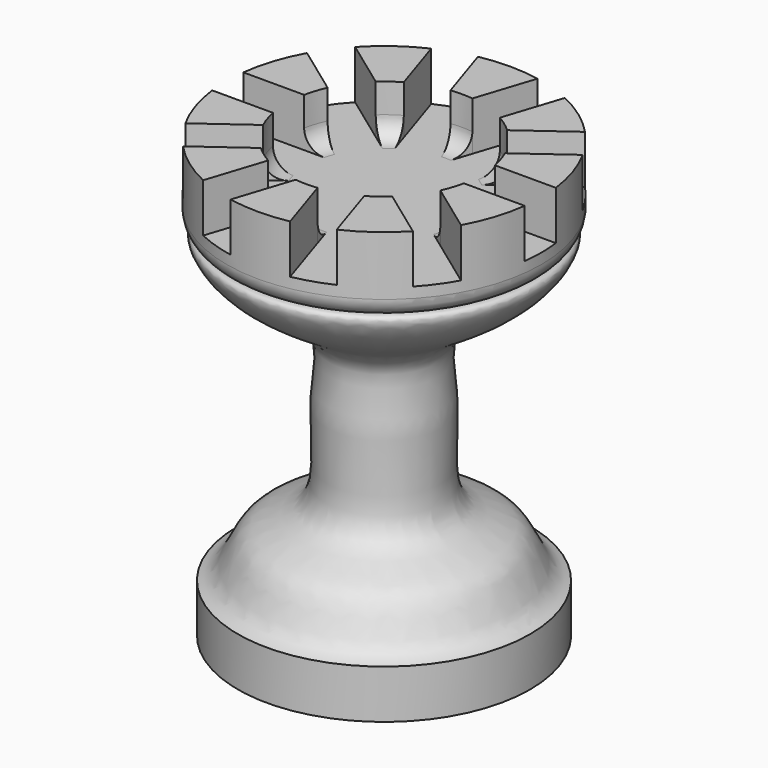
from build123d import *

# Parameters (mm, degrees)
F2_R          = 12.7
F3_DEPTH      = 6.35
F4_W          = 13.9516657994
F4_H          = 5.08
F5_DEPTH      = 6.35
F6_T4_ANGLE   = 70.2223360854
F6_T9_ANGLE   = 70.2223360854
F6_T15_ANGLE  = 70.2223360854
F6_T20_ANGLE  = 70.2223360854
F6_T25_ANGLE  = 70.2223360854
F6_T31_ANGLE  = 70.2223360854
F6_T36_ANGLE  = 70.2223360854
F6_T41_ANGLE  = 70.2223360854
F6_T47_ANGLE  = 70.2223360854
F6_T52_ANGLE  = 70.2223360854
F6_T57_ANGLE  = 70.2223360854
F6_T63_ANGLE  = 70.2223360854
F6_T68_ANGLE  = 70.2223360854
F6_T73_ANGLE  = 70.2223360854
F6_T79_ANGLE  = 70.2223360854
F6_T84_ANGLE  = 70.2223360854
F6_T89_ANGLE  = 70.2223360854
F6_T95_ANGLE  = 70.2223360854
F6_T100_ANGLE = 70.2223360854
F6_T105_ANGLE = 70.2223360854
F6_T111_ANGLE = 70.2223360854
F6_T116_ANGLE = 70.2223360854
F6_T121_ANGLE = 70.2223360854
F6_T127_ANGLE = 70.2223360854
F6_T132_ANGLE = 70.2223360854
F6_T137_ANGLE = 70.2223360854
F6_T143_ANGLE = 70.2223360854
F6_T148_ANGLE = 70.2223360854
F6_T153_ANGLE = 70.2223360854
F6_T159_ANGLE = 70.2223360854


# Not quite as in the source:
# - a fillet or chamfer that OpenCascade refuses, or shapes differently, is made with other operations: its cross-section is extruded or revolved along the edge and cut away or added


with BuildPart() as f1:
    # F0 (on Front) → F1 (revolve)
    with BuildSketch(Plane.XZ):
        Polygon((0, 56.9858625531), (0, 46.99), (19.1146062934, 46.99), (20.5274569789, 46.99), (20.5274569789, 56.9858625531), align=None)
        with BuildLine():
            Line((0, 46.99), (0, 0))
            Line((0, 0), (19.05, 0))
            Line((19.05, 0), (19.05, 6.35))
            add(Edge.make_bspline(
                [(19.05, 6.35), (16.5339762391, 6.9432851518), (16.0569680771, 13.155913981), (7.6273097689, 13.9182189792), (7.2848350223, 21.1697275176), (7.7653617057, 27.9522467214), (6.3029058207, 34.9075424246), (11.924104766, 38.4900940868), (18.9862936416, 42.8343809655), (20.5274569789, 46.99), (19.1146062934, 46.99)],
                knots=[0, 0, 0, 0, 0.1315490965, 0.2608144657, 0.383337474, 0.5182610911, 0.6426548645, 0.7643816563, 0.9167734046, 1, 1, 1, 1], degree=3))
            Line((19.1146062934, 46.99), (0, 46.99))
        make_face()
    revolve(axis=Axis((0, 0, 28.575), (0, 0, 1)))

    # F2 (on face) → F3 (cut)
    with BuildSketch(Plane.XY.offset(56.9858625531)):
        Circle(F2_R)
    extrude(amount=-F3_DEPTH, mode=Mode.SUBTRACT)

    # F4 (on face) → F5 (cut)
    with BuildSketch(Plane.XY.offset(56.9858625531)):
        with Locations((15.748, 0)):
            Rectangle(F4_W, F4_H)
        Polygon((8.5898068025, 3.1012472865), (19.876941534, 11.3018306883), (16.8909924524, 15.4116370197), (5.6038577208, 7.2110536179), align=None)
        Polygon((5.1264322629, 7.5579235171), (9.4377340947, 20.8267461887), (4.606366992, 22.3965525202), (0.2950651601, 9.1277298485), align=None)
        Polygon((-0.2950651601, 9.1277298485), (-4.606366992, 22.3965525202), (-9.4377340947, 20.8267461887), (-5.1264322629, 7.5579235171), align=None)
        Polygon((-5.6038577208, 7.2110536179), (-16.8909924524, 15.4116370197), (-19.876941534, 11.3018306883), (-8.5898068025, 3.1012472865), align=None)
        with Locations((-15.748, 0)):
            Rectangle(F4_W, F4_H)
        Polygon((-8.5898068025, -3.1012472865), (-19.876941534, -11.3018306883), (-16.8909924524, -15.4116370197), (-5.6038577208, -7.2110536179), align=None)
        Polygon((-5.1264322629, -7.5579235171), (-9.4377340947, -20.8267461887), (-4.606366992, -22.3965525202), (-0.2950651601, -9.1277298485), align=None)
        Polygon((0.2950651601, -9.1277298485), (4.606366992, -22.3965525202), (9.4377340947, -20.8267461887), (5.1264322629, -7.5579235171), align=None)
        Polygon((5.6038577208, -7.2110536179), (16.8909924524, -15.4116370197), (19.876941534, -11.3018306883), (8.5898068025, -3.1012472865), align=None)
    extrude(amount=-F5_DEPTH, mode=Mode.SUBTRACT)

    # F6: fillet of radius 2.54 on 11 edges, made by hand


with BuildPart() as f6_tool2:
    # F6_s3 → F6_t4 (revolve)
    with BuildSketch(Plane(origin=(0, 0, 0), x_dir=(0, 0, 1), z_dir=(-0.3237330019, 0.9461484786, 0))):
        with BuildLine():
            ThreePointArc((50.6358625531, -10.16), (51.3798113289, -11.9560512242), (53.1758625531, -12.7))
            Line((53.1758625531, -12.7), (50.6358625531, -12.7))
            Line((50.6358625531, -12.7), (50.6358625531, -10.16))
        make_face()
    revolve(axis=Axis((0, 0, 50.6358625531), (0, 0, 1)), revolution_arc=F6_T4_ANGLE)

    split(bisect_by=Plane(origin=(-1.4929745408, 2.0549031657, 0), x_dir=(0, 0, 1), z_dir=(-0.5877852523, 0.8090169944, 0)), keep=Keep.TOP)


with BuildPart() as f1_1:
    add(f1.part)

    # F6_t1: union F6_tool2
    add(f6_tool2.part)


with BuildPart() as f6_tool7:
    # F6_s8 → F6_t9 (revolve)
    with BuildSketch(Plane(origin=(0, 0, 0), x_dir=(0, 0, 1), z_dir=(-0.3237330019, 0.9461484786, 0))):
        with BuildLine():
            ThreePointArc((50.6358625531, -10.16), (51.3798113289, -11.9560512242), (53.1758625531, -12.7))
            Line((53.1758625531, -12.7), (50.6358625531, -12.7))
            Line((50.6358625531, -12.7), (50.6358625531, -10.16))
        make_face()
    revolve(axis=Axis((0, 0, 50.6358625531), (0, 0, 1)), revolution_arc=F6_T9_ANGLE)

    split(bisect_by=Plane(origin=(1.4929745408, -2.0549031657, 0), x_dir=(0, 0, 1), z_dir=(0.5877852523, -0.8090169944, 0)), keep=Keep.TOP)

    split(bisect_by=Plane(origin=(-2.4156835514, 0.7849031657, 0), x_dir=(0, 0, 1), z_dir=(-0.9510565163, 0.3090169944, 0)), keep=Keep.TOP)


with BuildPart() as f1_2:
    add(f1_1.part)

    # F6_t6: union F6_tool7
    add(f6_tool7.part)


with BuildPart() as f6_tool13:
    # F6_s14 → F6_t15 (revolve)
    with BuildSketch(Plane(origin=(0, 0, 0), x_dir=(0, 0, 1), z_dir=(-0.3237330019, 0.9461484786, 0))):
        with BuildLine():
            ThreePointArc((50.6358625531, -10.16), (51.3798113289, -11.9560512242), (53.1758625531, -12.7))
            Line((53.1758625531, -12.7), (50.6358625531, -12.7))
            Line((50.6358625531, -12.7), (50.6358625531, -10.16))
        make_face()
    revolve(axis=Axis((0, 0, 50.6358625531), (0, 0, 1)), revolution_arc=F6_T15_ANGLE)

    split(bisect_by=Plane(origin=(2.4156835514, -0.7849031657, 0), x_dir=(0, 0, 1), z_dir=(0.9510565163, -0.3090169944, 0)), keep=Keep.TOP)


with BuildPart() as f1_3:
    add(f1_2.part)

    # F6_t12: union F6_tool13
    add(f6_tool13.part)


with BuildPart() as f6_tool18:
    # F6_s19 → F6_t20 (revolve)
    with BuildSketch(Plane(origin=(0, 0, 0), x_dir=(0, 0, 1), z_dir=(0.294226622, 0.9557356826, 0))):
        with BuildLine():
            ThreePointArc((50.6358625531, -10.16), (51.3798113289, -11.9560512242), (53.1758625531, -12.7))
            Line((53.1758625531, -12.7), (50.6358625531, -12.7))
            Line((50.6358625531, -12.7), (50.6358625531, -10.16))
        make_face()
    revolve(axis=Axis((0, 0, 50.6358625531), (0, 0, 1)), revolution_arc=F6_T20_ANGLE)

    split(bisect_by=Plane.XZ.offset(-2.54), keep=Keep.BOTTOM)


with BuildPart() as f1_4:
    add(f1_3.part)

    # F6_t17: union F6_tool18
    add(f6_tool18.part)


with BuildPart() as f6_tool23:
    # F6_s24 → F6_t25 (revolve)
    with BuildSketch(Plane(origin=(0, 0, 0), x_dir=(0, 0, 1), z_dir=(0.294226622, 0.9557356826, 0))):
        with BuildLine():
            ThreePointArc((50.6358625531, -10.16), (51.3798113289, -11.9560512242), (53.1758625531, -12.7))
            Line((53.1758625531, -12.7), (50.6358625531, -12.7))
            Line((50.6358625531, -12.7), (50.6358625531, -10.16))
        make_face()
    revolve(axis=Axis((0, 0, 50.6358625531), (0, 0, 1)), revolution_arc=F6_T25_ANGLE)

    split(bisect_by=Plane.XZ.offset(2.54), keep=Keep.TOP)

    split(bisect_by=Plane(origin=(-1.4929745408, 2.0549031657, 0), x_dir=(0, 0, 1), z_dir=(-0.5877852523, 0.8090169944, 0)), keep=Keep.TOP)


with BuildPart() as f1_5:
    add(f1_4.part)

    # F6_t22: union F6_tool23
    add(f6_tool23.part)


with BuildPart() as f6_tool29:
    # F6_s30 → F6_t31 (revolve)
    with BuildSketch(Plane(origin=(0, 0, 0), x_dir=(0, 0, 1), z_dir=(0.294226622, 0.9557356826, 0))):
        with BuildLine():
            ThreePointArc((50.6358625531, -10.16), (51.3798113289, -11.9560512242), (53.1758625531, -12.7))
            Line((53.1758625531, -12.7), (50.6358625531, -12.7))
            Line((50.6358625531, -12.7), (50.6358625531, -10.16))
        make_face()
    revolve(axis=Axis((0, 0, 50.6358625531), (0, 0, 1)), revolution_arc=F6_T31_ANGLE)

    split(bisect_by=Plane(origin=(1.4929745408, -2.0549031657, 0), x_dir=(0, 0, 1), z_dir=(0.5877852523, -0.8090169944, 0)), keep=Keep.TOP)


with BuildPart() as f1_6:
    add(f1_5.part)

    # F6_t28: union F6_tool29
    add(f6_tool29.part)


with BuildPart() as f6_tool34:
    # F6_s35 → F6_t36 (revolve)
    with BuildSketch(Plane(origin=(0, 0, 0), x_dir=(0, 0, 1), z_dir=(0.7998016767, 0.6002643401, 0))):
        with BuildLine():
            ThreePointArc((50.6358625531, -10.16), (51.3798113289, -11.9560512242), (53.1758625531, -12.7))
            Line((53.1758625531, -12.7), (50.6358625531, -12.7))
            Line((50.6358625531, -12.7), (50.6358625531, -10.16))
        make_face()
    revolve(axis=Axis((0, 0, 50.6358625531), (0, 0, 1)), revolution_arc=F6_T36_ANGLE)

    split(bisect_by=Plane(origin=(1.4929745408, 2.0549031657, 0), x_dir=(0, 0, 1), z_dir=(0.5877852523, 0.8090169944, 0)), keep=Keep.TOP)


with BuildPart() as f1_7:
    add(f1_6.part)

    # F6_t33: union F6_tool34
    add(f6_tool34.part)


with BuildPart() as f6_tool39:
    # F6_s40 → F6_t41 (revolve)
    with BuildSketch(Plane(origin=(0, 0, 0), x_dir=(0, 0, 1), z_dir=(0.7998016767, 0.6002643401, 0))):
        with BuildLine():
            ThreePointArc((50.6358625531, -10.16), (51.3798113289, -11.9560512242), (53.1758625531, -12.7))
            Line((53.1758625531, -12.7), (50.6358625531, -12.7))
            Line((50.6358625531, -12.7), (50.6358625531, -10.16))
        make_face()
    revolve(axis=Axis((0, 0, 50.6358625531), (0, 0, 1)), revolution_arc=F6_T41_ANGLE)

    split(bisect_by=Plane(origin=(-1.4929745408, -2.0549031657, 0), x_dir=(0, 0, 1), z_dir=(-0.5877852523, -0.8090169944, 0)), keep=Keep.TOP)

    split(bisect_by=Plane.XZ.offset(-2.54), keep=Keep.BOTTOM)


with BuildPart() as f1_8:
    add(f1_7.part)

    # F6_t38: union F6_tool39
    add(f6_tool39.part)


with BuildPart() as f6_tool45:
    # F6_s46 → F6_t47 (revolve)
    with BuildSketch(Plane(origin=(0, 0, 0), x_dir=(0, 0, 1), z_dir=(0.7998016767, 0.6002643401, 0))):
        with BuildLine():
            ThreePointArc((50.6358625531, -10.16), (51.3798113289, -11.9560512242), (53.1758625531, -12.7))
            Line((53.1758625531, -12.7), (50.6358625531, -12.7))
            Line((50.6358625531, -12.7), (50.6358625531, -10.16))
        make_face()
    revolve(axis=Axis((0, 0, 50.6358625531), (0, 0, 1)), revolution_arc=F6_T47_ANGLE)

    split(bisect_by=Plane.XZ.offset(2.54), keep=Keep.TOP)


with BuildPart() as f1_9:
    add(f1_8.part)

    # F6_t44: union F6_tool45
    add(f6_tool45.part)


with BuildPart() as f6_tool50:
    # F6_s51 → F6_t52 (revolve)
    with BuildSketch(Plane(origin=(0, 0, 0), x_dir=(0, 0, 1), z_dir=(-0.8180376224, 0.5751647141, 0))):
        with BuildLine():
            ThreePointArc((50.6358625531, -10.16), (51.3798113289, -11.9560512242), (53.1758625531, -12.7))
            Line((53.1758625531, -12.7), (50.6358625531, -12.7))
            Line((50.6358625531, -12.7), (50.6358625531, -10.16))
        make_face()
    revolve(axis=Axis((0, 0, 50.6358625531), (0, 0, 1)), revolution_arc=F6_T52_ANGLE)

    split(bisect_by=Plane(origin=(-2.4156835514, 0.7849031657, 0), x_dir=(0, 0, 1), z_dir=(-0.9510565163, 0.3090169944, 0)), keep=Keep.TOP)


with BuildPart() as f1_10:
    add(f1_9.part)

    # F6_t49: union F6_tool50
    add(f6_tool50.part)


with BuildPart() as f6_tool55:
    # F6_s56 → F6_t57 (revolve)
    with BuildSketch(Plane(origin=(0, 0, 0), x_dir=(0, 0, 1), z_dir=(-0.8180376224, 0.5751647141, 0))):
        with BuildLine():
            ThreePointArc((50.6358625531, -10.16), (51.3798113289, -11.9560512242), (53.1758625531, -12.7))
            Line((53.1758625531, -12.7), (50.6358625531, -12.7))
            Line((50.6358625531, -12.7), (50.6358625531, -10.16))
        make_face()
    revolve(axis=Axis((0, 0, 50.6358625531), (0, 0, 1)), revolution_arc=F6_T57_ANGLE)

    split(bisect_by=Plane(origin=(2.4156835514, -0.7849031657, 0), x_dir=(0, 0, 1), z_dir=(0.9510565163, -0.3090169944, 0)), keep=Keep.TOP)

    split(bisect_by=Plane(origin=(-2.4156835514, -0.7849031657, 0), x_dir=(0, 0, 1), z_dir=(-0.9510565163, -0.3090169944, 0)), keep=Keep.TOP)


with BuildPart() as f1_11:
    add(f1_10.part)

    # F6_t54: union F6_tool55
    add(f6_tool55.part)


with BuildPart() as f6_tool61:
    # F6_s62 → F6_t63 (revolve)
    with BuildSketch(Plane(origin=(0, 0, 0), x_dir=(0, 0, 1), z_dir=(-0.8180376224, 0.5751647141, 0))):
        with BuildLine():
            ThreePointArc((50.6358625531, -10.16), (51.3798113289, -11.9560512242), (53.1758625531, -12.7))
            Line((53.1758625531, -12.7), (50.6358625531, -12.7))
            Line((50.6358625531, -12.7), (50.6358625531, -10.16))
        make_face()
    revolve(axis=Axis((0, 0, 50.6358625531), (0, 0, 1)), revolution_arc=F6_T63_ANGLE)

    split(bisect_by=Plane(origin=(2.4156835514, 0.7849031657, 0), x_dir=(0, 0, 1), z_dir=(0.9510565163, 0.3090169944, 0)), keep=Keep.TOP)


with BuildPart() as f1_12:
    add(f1_11.part)

    # F6_t60: union F6_tool61
    add(f6_tool61.part)


with BuildPart() as f6_tool66:
    # F6_s67 → F6_t68 (revolve)
    with BuildSketch(Plane(origin=(0, 0, 0), x_dir=(0, 0, 1), z_dir=(-0.9998796751, -0.0155124219, 0))):
        with BuildLine():
            ThreePointArc((50.6358625531, -10.16), (51.3798113289, -11.9560512242), (53.1758625531, -12.7))
            Line((53.1758625531, -12.7), (50.6358625531, -12.7))
            Line((50.6358625531, -12.7), (50.6358625531, -10.16))
        make_face()
    revolve(axis=Axis((0, 0, 50.6358625531), (0, 0, 1)), revolution_arc=F6_T68_ANGLE)

    split(bisect_by=Plane(origin=(-2.4156835514, -0.7849031657, 0), x_dir=(0, 0, 1), z_dir=(-0.9510565163, -0.3090169944, 0)), keep=Keep.TOP)


with BuildPart() as f1_13:
    add(f1_12.part)

    # F6_t65: union F6_tool66
    add(f6_tool66.part)


with BuildPart() as f6_tool71:
    # F6_s72 → F6_t73 (revolve)
    with BuildSketch(Plane(origin=(0, 0, 0), x_dir=(0, 0, 1), z_dir=(-0.9998796751, -0.0155124219, 0))):
        with BuildLine():
            ThreePointArc((50.6358625531, -10.16), (51.3798113289, -11.9560512242), (53.1758625531, -12.7))
            Line((53.1758625531, -12.7), (50.6358625531, -12.7))
            Line((50.6358625531, -12.7), (50.6358625531, -10.16))
        make_face()
    revolve(axis=Axis((0, 0, 50.6358625531), (0, 0, 1)), revolution_arc=F6_T73_ANGLE)

    split(bisect_by=Plane(origin=(2.4156835514, 0.7849031657, 0), x_dir=(0, 0, 1), z_dir=(0.9510565163, 0.3090169944, 0)), keep=Keep.TOP)

    split(bisect_by=Plane(origin=(-1.4929745408, -2.0549031657, 0), x_dir=(0, 0, 1), z_dir=(-0.5877852523, -0.8090169944, 0)), keep=Keep.TOP)


with BuildPart() as f1_14:
    add(f1_13.part)

    # F6_t70: union F6_tool71
    add(f6_tool71.part)


with BuildPart() as f6_tool77:
    # F6_s78 → F6_t79 (revolve)
    with BuildSketch(Plane(origin=(0, 0, 0), x_dir=(0, 0, 1), z_dir=(-0.9998796751, -0.0155124219, 0))):
        with BuildLine():
            ThreePointArc((50.6358625531, -10.16), (51.3798113289, -11.9560512242), (53.1758625531, -12.7))
            Line((53.1758625531, -12.7), (50.6358625531, -12.7))
            Line((50.6358625531, -12.7), (50.6358625531, -10.16))
        make_face()
    revolve(axis=Axis((0, 0, 50.6358625531), (0, 0, 1)), revolution_arc=F6_T79_ANGLE)

    split(bisect_by=Plane(origin=(1.4929745408, 2.0549031657, 0), x_dir=(0, 0, 1), z_dir=(0.5877852523, 0.8090169944, 0)), keep=Keep.TOP)


with BuildPart() as f1_15:
    add(f1_14.part)

    # F6_t76: union F6_tool77
    add(f6_tool77.part)


with BuildPart() as f6_tool82:
    # F6_s83 → F6_t84 (revolve)
    with BuildSketch(Plane(origin=(0, 0, 0), x_dir=(0, 0, 1), z_dir=(-0.7998016767, -0.6002643401, 0))):
        with BuildLine():
            ThreePointArc((50.6358625531, -10.16), (51.3798113289, -11.9560512242), (53.1758625531, -12.7))
            Line((53.1758625531, -12.7), (50.6358625531, -12.7))
            Line((50.6358625531, -12.7), (50.6358625531, -10.16))
        make_face()
    revolve(axis=Axis((0, 0, 50.6358625531), (0, 0, 1)), revolution_arc=F6_T84_ANGLE)

    split(bisect_by=Plane(origin=(-1.4929745408, -2.0549031657, 0), x_dir=(0, 0, 1), z_dir=(-0.5877852523, -0.8090169944, 0)), keep=Keep.TOP)


with BuildPart() as f1_16:
    add(f1_15.part)

    # F6_t81: union F6_tool82
    add(f6_tool82.part)


with BuildPart() as f6_tool87:
    # F6_s88 → F6_t89 (revolve)
    with BuildSketch(Plane(origin=(0, 0, 0), x_dir=(0, 0, 1), z_dir=(-0.7998016767, -0.6002643401, 0))):
        with BuildLine():
            ThreePointArc((50.6358625531, -10.16), (51.3798113289, -11.9560512242), (53.1758625531, -12.7))
            Line((53.1758625531, -12.7), (50.6358625531, -12.7))
            Line((50.6358625531, -12.7), (50.6358625531, -10.16))
        make_face()
    revolve(axis=Axis((0, 0, 50.6358625531), (0, 0, 1)), revolution_arc=F6_T89_ANGLE)

    split(bisect_by=Plane(origin=(1.4929745408, 2.0549031657, 0), x_dir=(0, 0, 1), z_dir=(0.5877852523, 0.8090169944, 0)), keep=Keep.TOP)

    split(bisect_by=Plane.XZ.offset(2.54), keep=Keep.TOP)


with BuildPart() as f1_17:
    add(f1_16.part)

    # F6_t86: union F6_tool87
    add(f6_tool87.part)


with BuildPart() as f6_tool93:
    # F6_s94 → F6_t95 (revolve)
    with BuildSketch(Plane(origin=(0, 0, 0), x_dir=(0, 0, 1), z_dir=(-0.7998016767, -0.6002643401, 0))):
        with BuildLine():
            ThreePointArc((50.6358625531, -10.16), (51.3798113289, -11.9560512242), (53.1758625531, -12.7))
            Line((53.1758625531, -12.7), (50.6358625531, -12.7))
            Line((50.6358625531, -12.7), (50.6358625531, -10.16))
        make_face()
    revolve(axis=Axis((0, 0, 50.6358625531), (0, 0, 1)), revolution_arc=F6_T95_ANGLE)

    split(bisect_by=Plane.XZ.offset(-2.54), keep=Keep.BOTTOM)


with BuildPart() as f1_18:
    add(f1_17.part)

    # F6_t92: union F6_tool93
    add(f6_tool93.part)


with BuildPart() as f6_tool98:
    # F6_s99 → F6_t100 (revolve)
    with BuildSketch(Plane(origin=(0, 0, 0), x_dir=(0, 0, 1), z_dir=(-0.294226622, -0.9557356826, 0))):
        with BuildLine():
            ThreePointArc((50.6358625531, -10.16), (51.3798113289, -11.9560512242), (53.1758625531, -12.7))
            Line((53.1758625531, -12.7), (50.6358625531, -12.7))
            Line((50.6358625531, -12.7), (50.6358625531, -10.16))
        make_face()
    revolve(axis=Axis((0, 0, 50.6358625531), (0, 0, 1)), revolution_arc=F6_T100_ANGLE)

    split(bisect_by=Plane.XZ.offset(2.54), keep=Keep.TOP)


with BuildPart() as f1_19:
    add(f1_18.part)

    # F6_t97: union F6_tool98
    add(f6_tool98.part)


with BuildPart() as f6_tool103:
    # F6_s104 → F6_t105 (revolve)
    with BuildSketch(Plane(origin=(0, 0, 0), x_dir=(0, 0, 1), z_dir=(-0.294226622, -0.9557356826, 0))):
        with BuildLine():
            ThreePointArc((50.6358625531, -10.16), (51.3798113289, -11.9560512242), (53.1758625531, -12.7))
            Line((53.1758625531, -12.7), (50.6358625531, -12.7))
            Line((50.6358625531, -12.7), (50.6358625531, -10.16))
        make_face()
    revolve(axis=Axis((0, 0, 50.6358625531), (0, 0, 1)), revolution_arc=F6_T105_ANGLE)

    split(bisect_by=Plane.XZ.offset(-2.54), keep=Keep.BOTTOM)

    split(bisect_by=Plane(origin=(1.4929745408, -2.0549031657, 0), x_dir=(0, 0, 1), z_dir=(0.5877852523, -0.8090169944, 0)), keep=Keep.TOP)


with BuildPart() as f1_20:
    add(f1_19.part)

    # F6_t102: union F6_tool103
    add(f6_tool103.part)


with BuildPart() as f6_tool109:
    # F6_s110 → F6_t111 (revolve)
    with BuildSketch(Plane(origin=(0, 0, 0), x_dir=(0, 0, 1), z_dir=(-0.294226622, -0.9557356826, 0))):
        with BuildLine():
            ThreePointArc((50.6358625531, -10.16), (51.3798113289, -11.9560512242), (53.1758625531, -12.7))
            Line((53.1758625531, -12.7), (50.6358625531, -12.7))
            Line((50.6358625531, -12.7), (50.6358625531, -10.16))
        make_face()
    revolve(axis=Axis((0, 0, 50.6358625531), (0, 0, 1)), revolution_arc=F6_T111_ANGLE)

    split(bisect_by=Plane(origin=(-1.4929745408, 2.0549031657, 0), x_dir=(0, 0, 1), z_dir=(-0.5877852523, 0.8090169944, 0)), keep=Keep.TOP)


with BuildPart() as f1_21:
    add(f1_20.part)

    # F6_t108: union F6_tool109
    add(f6_tool109.part)


with BuildPart() as f6_tool114:
    # F6_s115 → F6_t116 (revolve)
    with BuildSketch(Plane(origin=(0, 0, 0), x_dir=(0, 0, 1), z_dir=(0.3237330019, -0.9461484786, 0))):
        with BuildLine():
            ThreePointArc((50.6358625531, -10.16), (51.3798113289, -11.9560512242), (53.1758625531, -12.7))
            Line((53.1758625531, -12.7), (50.6358625531, -12.7))
            Line((50.6358625531, -12.7), (50.6358625531, -10.16))
        make_face()
    revolve(axis=Axis((0, 0, 50.6358625531), (0, 0, 1)), revolution_arc=F6_T116_ANGLE)

    split(bisect_by=Plane(origin=(1.4929745408, -2.0549031657, 0), x_dir=(0, 0, 1), z_dir=(0.5877852523, -0.8090169944, 0)), keep=Keep.TOP)


with BuildPart() as f1_22:
    add(f1_21.part)

    # F6_t113: union F6_tool114
    add(f6_tool114.part)


with BuildPart() as f6_tool119:
    # F6_s120 → F6_t121 (revolve)
    with BuildSketch(Plane(origin=(0, 0, 0), x_dir=(0, 0, 1), z_dir=(0.3237330019, -0.9461484786, 0))):
        with BuildLine():
            ThreePointArc((50.6358625531, -10.16), (51.3798113289, -11.9560512242), (53.1758625531, -12.7))
            Line((53.1758625531, -12.7), (50.6358625531, -12.7))
            Line((50.6358625531, -12.7), (50.6358625531, -10.16))
        make_face()
    revolve(axis=Axis((0, 0, 50.6358625531), (0, 0, 1)), revolution_arc=F6_T121_ANGLE)

    split(bisect_by=Plane(origin=(-1.4929745408, 2.0549031657, 0), x_dir=(0, 0, 1), z_dir=(-0.5877852523, 0.8090169944, 0)), keep=Keep.TOP)

    split(bisect_by=Plane(origin=(2.4156835514, -0.7849031657, 0), x_dir=(0, 0, 1), z_dir=(0.9510565163, -0.3090169944, 0)), keep=Keep.TOP)


with BuildPart() as f1_23:
    add(f1_22.part)

    # F6_t118: union F6_tool119
    add(f6_tool119.part)


with BuildPart() as f6_tool125:
    # F6_s126 → F6_t127 (revolve)
    with BuildSketch(Plane(origin=(0, 0, 0), x_dir=(0, 0, 1), z_dir=(0.3237330019, -0.9461484786, 0))):
        with BuildLine():
            ThreePointArc((50.6358625531, -10.16), (51.3798113289, -11.9560512242), (53.1758625531, -12.7))
            Line((53.1758625531, -12.7), (50.6358625531, -12.7))
            Line((50.6358625531, -12.7), (50.6358625531, -10.16))
        make_face()
    revolve(axis=Axis((0, 0, 50.6358625531), (0, 0, 1)), revolution_arc=F6_T127_ANGLE)

    split(bisect_by=Plane(origin=(-2.4156835514, 0.7849031657, 0), x_dir=(0, 0, 1), z_dir=(-0.9510565163, 0.3090169944, 0)), keep=Keep.TOP)


with BuildPart() as f1_24:
    add(f1_23.part)

    # F6_t124: union F6_tool125
    add(f6_tool125.part)


with BuildPart() as f6_tool130:
    # F6_s131 → F6_t132 (revolve)
    with BuildSketch(Plane(origin=(0, 0, 0), x_dir=(0, 0, 1), z_dir=(0.9998796751, 0.0155124219, 0))):
        with BuildLine():
            ThreePointArc((50.6358625531, -10.16), (51.3798113289, -11.9560512242), (53.1758625531, -12.7))
            Line((53.1758625531, -12.7), (50.6358625531, -12.7))
            Line((50.6358625531, -12.7), (50.6358625531, -10.16))
        make_face()
    revolve(axis=Axis((0, 0, 50.6358625531), (0, 0, 1)), revolution_arc=F6_T132_ANGLE)

    split(bisect_by=Plane(origin=(2.4156835514, 0.7849031657, 0), x_dir=(0, 0, 1), z_dir=(0.9510565163, 0.3090169944, 0)), keep=Keep.TOP)


with BuildPart() as f1_25:
    add(f1_24.part)

    # F6_t129: union F6_tool130
    add(f6_tool130.part)


with BuildPart() as f6_tool135:
    # F6_s136 → F6_t137 (revolve)
    with BuildSketch(Plane(origin=(0, 0, 0), x_dir=(0, 0, 1), z_dir=(0.9998796751, 0.0155124219, 0))):
        with BuildLine():
            ThreePointArc((50.6358625531, -10.16), (51.3798113289, -11.9560512242), (53.1758625531, -12.7))
            Line((53.1758625531, -12.7), (50.6358625531, -12.7))
            Line((50.6358625531, -12.7), (50.6358625531, -10.16))
        make_face()
    revolve(axis=Axis((0, 0, 50.6358625531), (0, 0, 1)), revolution_arc=F6_T137_ANGLE)

    split(bisect_by=Plane(origin=(-2.4156835514, -0.7849031657, 0), x_dir=(0, 0, 1), z_dir=(-0.9510565163, -0.3090169944, 0)), keep=Keep.TOP)

    split(bisect_by=Plane(origin=(1.4929745408, 2.0549031657, 0), x_dir=(0, 0, 1), z_dir=(0.5877852523, 0.8090169944, 0)), keep=Keep.TOP)


with BuildPart() as f1_26:
    add(f1_25.part)

    # F6_t134: union F6_tool135
    add(f6_tool135.part)


with BuildPart() as f6_tool141:
    # F6_s142 → F6_t143 (revolve)
    with BuildSketch(Plane(origin=(0, 0, 0), x_dir=(0, 0, 1), z_dir=(0.9998796751, 0.0155124219, 0))):
        with BuildLine():
            ThreePointArc((50.6358625531, -10.16), (51.3798113289, -11.9560512242), (53.1758625531, -12.7))
            Line((53.1758625531, -12.7), (50.6358625531, -12.7))
            Line((50.6358625531, -12.7), (50.6358625531, -10.16))
        make_face()
    revolve(axis=Axis((0, 0, 50.6358625531), (0, 0, 1)), revolution_arc=F6_T143_ANGLE)

    split(bisect_by=Plane(origin=(-1.4929745408, -2.0549031657, 0), x_dir=(0, 0, 1), z_dir=(-0.5877852523, -0.8090169944, 0)), keep=Keep.TOP)


with BuildPart() as f1_27:
    add(f1_26.part)

    # F6_t140: union F6_tool141
    add(f6_tool141.part)


with BuildPart() as f6_tool146:
    # F6_s147 → F6_t148 (revolve)
    with BuildSketch(Plane(origin=(0, 0, 0), x_dir=(0, 0, 1), z_dir=(0.8180376224, -0.5751647141, 0))):
        with BuildLine():
            ThreePointArc((50.6358625531, -10.16), (51.3798113289, -11.9560512242), (53.1758625531, -12.7))
            Line((53.1758625531, -12.7), (50.6358625531, -12.7))
            Line((50.6358625531, -12.7), (50.6358625531, -10.16))
        make_face()
    revolve(axis=Axis((0, 0, 50.6358625531), (0, 0, 1)), revolution_arc=F6_T148_ANGLE)

    split(bisect_by=Plane(origin=(2.4156835514, -0.7849031657, 0), x_dir=(0, 0, 1), z_dir=(0.9510565163, -0.3090169944, 0)), keep=Keep.TOP)


with BuildPart() as f1_28:
    add(f1_27.part)

    # F6_t145: union F6_tool146
    add(f6_tool146.part)


with BuildPart() as f6_tool151:
    # F6_s152 → F6_t153 (revolve)
    with BuildSketch(Plane(origin=(0, 0, 0), x_dir=(0, 0, 1), z_dir=(0.8180376224, -0.5751647141, 0))):
        with BuildLine():
            ThreePointArc((50.6358625531, -10.16), (51.3798113289, -11.9560512242), (53.1758625531, -12.7))
            Line((53.1758625531, -12.7), (50.6358625531, -12.7))
            Line((50.6358625531, -12.7), (50.6358625531, -10.16))
        make_face()
    revolve(axis=Axis((0, 0, 50.6358625531), (0, 0, 1)), revolution_arc=F6_T153_ANGLE)

    split(bisect_by=Plane(origin=(-2.4156835514, 0.7849031657, 0), x_dir=(0, 0, 1), z_dir=(-0.9510565163, 0.3090169944, 0)), keep=Keep.TOP)

    split(bisect_by=Plane(origin=(2.4156835514, 0.7849031657, 0), x_dir=(0, 0, 1), z_dir=(0.9510565163, 0.3090169944, 0)), keep=Keep.TOP)


with BuildPart() as f1_29:
    add(f1_28.part)

    # F6_t150: union F6_tool151
    add(f6_tool151.part)


with BuildPart() as f6_tool157:
    # F6_s158 → F6_t159 (revolve)
    with BuildSketch(Plane(origin=(0, 0, 0), x_dir=(0, 0, 1), z_dir=(0.8180376224, -0.5751647141, 0))):
        with BuildLine():
            ThreePointArc((50.6358625531, -10.16), (51.3798113289, -11.9560512242), (53.1758625531, -12.7))
            Line((53.1758625531, -12.7), (50.6358625531, -12.7))
            Line((50.6358625531, -12.7), (50.6358625531, -10.16))
        make_face()
    revolve(axis=Axis((0, 0, 50.6358625531), (0, 0, 1)), revolution_arc=F6_T159_ANGLE)

    split(bisect_by=Plane(origin=(-2.4156835514, -0.7849031657, 0), x_dir=(0, 0, 1), z_dir=(-0.9510565163, -0.3090169944, 0)), keep=Keep.TOP)


with BuildPart() as f1_30:
    add(f1_29.part)

    # F6_t156: union F6_tool157
    add(f6_tool157.part)

    # F6_s161 → F6_t162 (revolve, cut)
    with BuildSketch(Plane.XZ):
        with BuildLine():
            ThreePointArc((19.1146062934, 46.99), (20.1455301077, 47.9266880989), (20.5274569789, 49.2662105401))
            Line((20.5274569789, 49.2662105401), (20.5274569789, 46.99))
            Line((20.5274569789, 46.99), (19.1146062934, 46.99))
        make_face()
    revolve(axis=Axis((0, 0, 46.99), (0, 0, 1)), mode=Mode.SUBTRACT)


solid = f1_30.part
